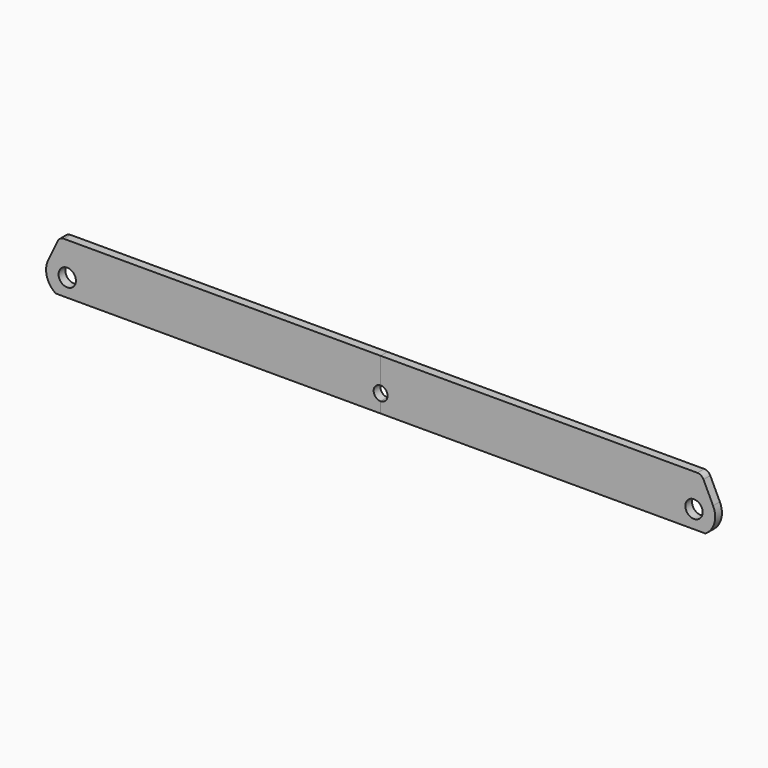
from build123d import *
from build123d import SkipClean  # not in build123d's __all__

# Parameters (mm, degrees)
F0_R     = 5.125
F1_DEPTH = 5


with BuildPart() as f1:
    # F0 (on Front) → F1 (new body)
    with BuildSketch(Plane.XZ):
        with BuildLine():
            Line((-191.7823299831, 0), (0, 0))
            Line((0, 0), (0, 6.375))
            ThreePointArc((0, 6.375), (-4.125, 10.5), (0, 14.625))
            Line((0, 14.625), (0, 30))
            Line((0, 30), (-187, 30))
            ThreePointArc((-187, 30), (-189.1316333954, 29.3846918719), (-190.6074611137, 27.7280695337))
            Line((-190.6074611137, 27.7280695337), (-196.2733159802, 15.9002172929))
            ThreePointArc((-196.2733159802, 15.9002172929), (-197.029373021, 7.1023265723), (-191.7823299831, 0))
        make_face()
        with Locations((-185, 10.5)):
            Circle(F0_R, mode=Mode.SUBTRACT)
    extrude(amount=F1_DEPTH)

    # F2: F1 across plane


with BuildPart() as f1_1:
    add(f1.part, clean=False)
    with SkipClean():  # cleaning this boolean's faces spoils the solid; the shape is the same uncleaned
        add(f1.part.mirror(Plane.YZ), clean=False)


solid = f1_1.part
